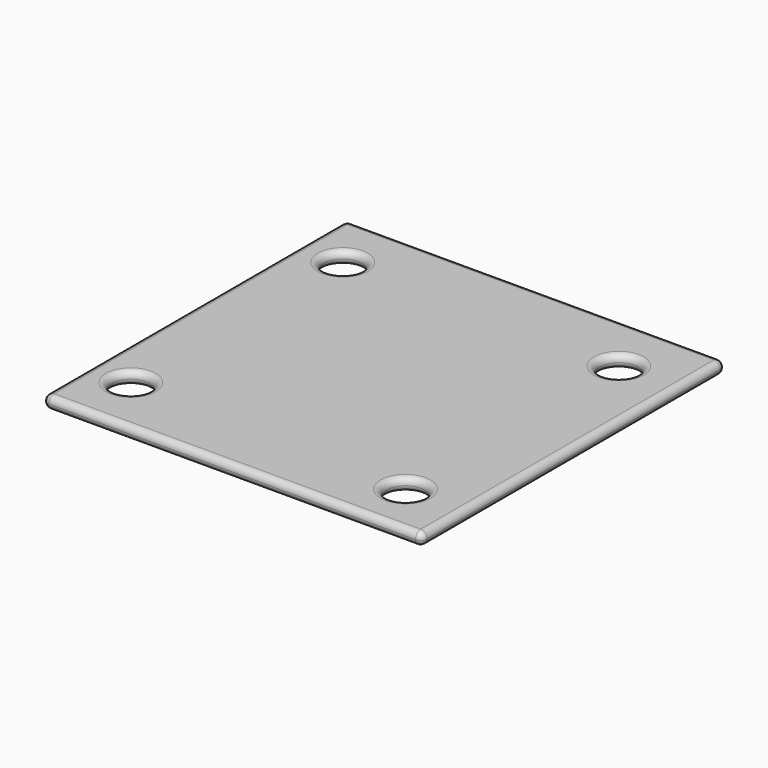
from build123d import *

# Parameters (mm, degrees)
F0_W     = 30
F0_H     = 30
F0_R     = 1.5
F1_DEPTH = 1
F1_TAPER = -3
F2_R     = 0.4999
F3_R     = 0.49999


# Not quite as in the source:
# - a fillet or chamfer is up to 0.001 mm smaller than in the source, because OpenCascade refuses the exact size


with BuildPart() as f1:
    # F0 (on Top) → F1 (new body)
    with BuildSketch(Plane.XY):
        Rectangle(F0_W, F0_H)
        with Locations((-11.7577761412, -10.388918221)):
            Circle(F0_R, mode=Mode.SUBTRACT)
        with Locations((10.4432478547, -10.9203271568)):
            Circle(F0_R, mode=Mode.SUBTRACT)
        with Locations((-11.5806385875, 10.3950165212)):
            Circle(F0_R, mode=Mode.SUBTRACT)
        with Locations((10.4432478547, 10.2178789675)):
            Circle(F0_R, mode=Mode.SUBTRACT)
    extrude(amount=F1_DEPTH, taper=F1_TAPER)

    # F2 (radius 0.5 in the source; OpenCascade refuses exactly that, so slightly less here)
    f2_edges = [f1.edges().sort_by_distance(p)[0] for p in [
        (0, -15.052408, 1),
        (0, -15, 0),
        (-15, 0, 0),
        (-15.052408, 0, 1),
        (15.052408, 0, 1),
        (0, 15.052408, 1),
        (0, 15, 0),
        (15, 0, 0),
        (-15.026204, -15.026204, 0.5),
        (15.026204, -15.026204, 0.5),
        (-15.026204, 15.026204, 0.5),
        (15.026204, 15.026204, 0.5),
    ]]
    fillet(f2_edges, radius=F2_R)

    # F3 (radius 0.5 in the source; OpenCascade refuses exactly that, so slightly less here)
    f3_edges = [f1.edges().sort_by_distance(p)[0] for p in [
        (8.995656, -10.920327, 1),
        (-13.205368, -10.388918, 1),
        (-13.028231, 10.395017, 1),
        (8.995656, 10.217879, 1),
        (8.943248, -10.920327, 0),
        (-13.257776, -10.388918, 0),
        (-13.080639, 10.395017, 0),
        (8.943248, 10.217879, 0),
    ]]
    fillet(f3_edges, radius=F3_R)


solid = f1.part
